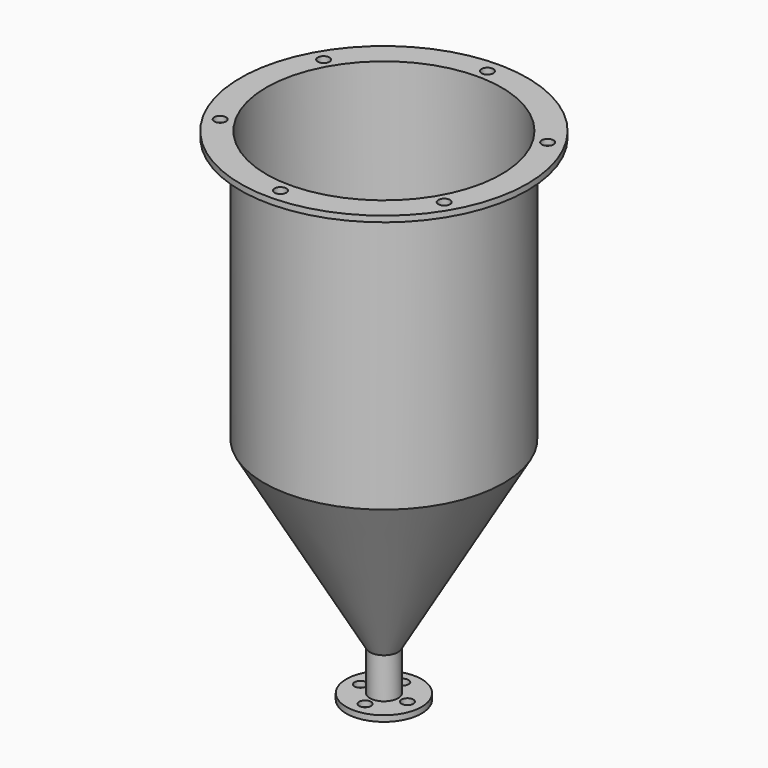
from build123d import *

# Parameters (mm, degrees)
F2_R     = 122
F2_R_2   = 102
F3_DEPTH = 5
F4_R     = 32
F4_R_2   = 12
F5_DEPTH = 5
F6_R     = 5
F7_DEPTH = 425.8855726812
F8_R     = 5
F9_DEPTH = 5


with BuildPart() as f1:
    # F0 (on Front) → F1 (revolve)
    with BuildSketch(Plane.XZ):
        Polygon((-100, 195.8845726812), (-100, 425.8845726812), (-102, 425.8845726812), (-102, 195.3486742963), (-12, 39.4641016151), (-12, 0), (-10, 0), (-10, 40), align=None)
    revolve(axis=Axis((0, 0, 212.9422863406), (0, 0, 1)))

    # F2 (on face) → F3 (join)
    with BuildSketch(Plane.XY.offset(425.8845726812)):
        Circle(F2_R)
        Circle(F2_R_2, mode=Mode.SUBTRACT)
    extrude(amount=-F3_DEPTH)

    # F4 (on face) → F5 (join)
    with BuildSketch(Plane(origin=(0, 0, 0), x_dir=(1, 0, 0), z_dir=(0, 0, -1))):
        Circle(F4_R)
        Circle(F4_R_2, mode=Mode.SUBTRACT)
    extrude(amount=-F5_DEPTH)

    # F6 (on face) → F7 (cut, through all)
    with BuildSketch(Plane.XY.offset(425.8845726812)):
        with Locations((0, 110)):
            Circle(F6_R)
        with Locations((-95.2627944163, 55)):
            Circle(F6_R)
        with Locations((-95.2627944163, -55)):
            Circle(F6_R)
        with Locations((0, -110)):
            Circle(F6_R)
        with Locations((95.2627944163, -55)):
            Circle(F6_R)
        with Locations((95.2627944163, 55)):
            Circle(F6_R)
    extrude(amount=-F7_DEPTH, mode=Mode.SUBTRACT)

    # F8 (on face) → F9 (cut, through all)
    with BuildSketch(Plane(origin=(0, 0, 0), x_dir=(1, 0, 0), z_dir=(0, 0, -1))):
        with Locations((0, 20)):
            Circle(F8_R)
        with Locations((-20, 0)):
            Circle(F8_R)
        with Locations((0, -20)):
            Circle(F8_R)
        with Locations((20, 0)):
            Circle(F8_R)
    extrude(amount=-F9_DEPTH, mode=Mode.SUBTRACT)


solid = f1.part
